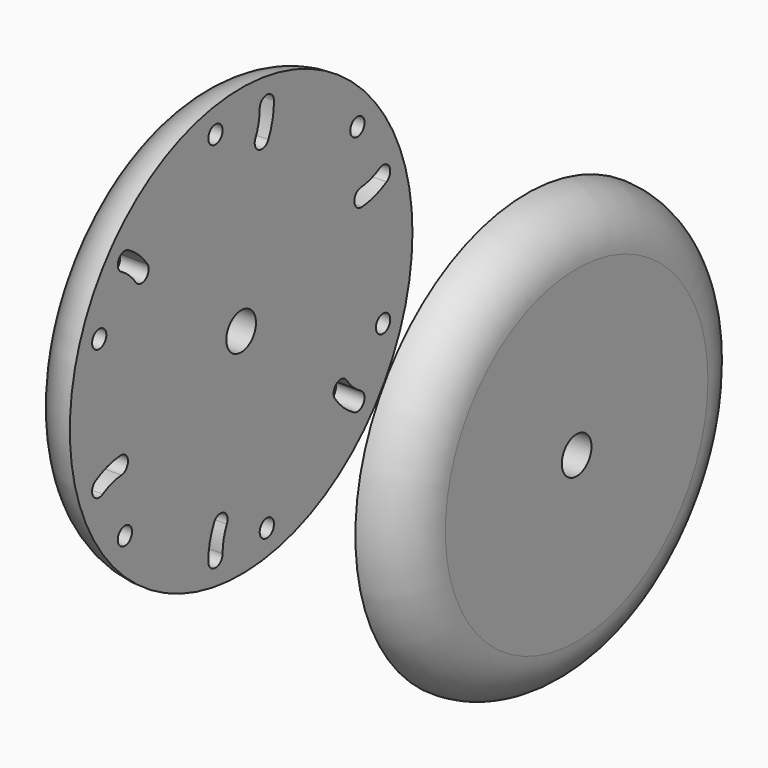
from build123d import *

# Parameters (mm, degrees)
F0_R     = 38.1
F1_DEPTH = 8.89
F2_R     = 8.88999
F3_R     = 3.302
F4_DEPTH = 8.89
F5_R     = 1.5875
F6_DEPTH = 5.08


# Not quite as in the source:
# - a fillet or chamfer is up to 0.001 mm smaller than in the source, because OpenCascade refuses the exact size


with BuildPart() as f1:
    # F0 (on Right) → F1 (new body)
    with BuildSketch(Plane.YZ):
        Circle(F0_R)
    extrude(amount=F1_DEPTH)

    # F2 (radius 8.89 in the source; OpenCascade refuses exactly that, so slightly less here)
    f2_edges = [f1.edges().sort_by_distance(p)[0] for p in [
        (8.89, -38.1, 0),
    ]]
    fillet(f2_edges, radius=F2_R)

    # F3 (on face) → F4 (cut)
    with BuildSketch(Plane.YZ.offset(8.89)):
        Circle(F3_R)
    extrude(amount=-F4_DEPTH, mode=Mode.SUBTRACT)

    # F5 (on face) → F6 (cut)
    with BuildSketch(Plane(origin=(0, 0, 0), x_dir=(0, -1, 0), z_dir=(-1, 0, 0))):
        with Locations((5.715, 33.1496630312)):
            Circle(F5_R)
        with BuildLine():
            ThreePointArc((-5.6047569444, 31.5659955413), (-4.5541453363, 32.0668090708), (-4.1275, 33.1496630312))
            ThreePointArc((-4.1275, 33.1496630312), (-5.715, 34.7371630312), (-7.3025, 33.1496630312))
            ThreePointArc((-7.3025, 33.1496630312), (-6.7978539604, 31.9888083675), (-5.6047569444, 31.5659955413))
        make_face()
        with BuildLine():
            ThreePointArc((-3.1712978707, 28.9178175232), (-3.8854737654, 30.9803982412), (-4.1275, 33.1496630312))
            ThreePointArc((-4.1275, 33.1496630312), (-4.5541453363, 32.0668090708), (-5.6047569444, 31.5659955413))
            ThreePointArc((-5.6047569444, 31.5659955413), (-5.433937276, 30.6305168235), (-5.1859467295, 29.712475169))
            ThreePointArc((-5.1859467295, 29.712475169), (-4.0220744225, 29.712032986), (-3.1712978707, 28.9178175232))
        make_face()
        with BuildLine():
            ThreePointArc((-5.6047569444, 31.5659955413), (-6.7978539604, 31.9888083675), (-7.3025, 33.1496630312))
            ThreePointArc((-7.3025, 33.1496630312), (-6.9824007866, 30.2806354058), (-6.0378455709, 27.552706069))
            ThreePointArc((-6.0378455709, 27.552706069), (-6.0813429107, 28.8177590943), (-5.1859467295, 29.712475169))
            ThreePointArc((-5.1859467295, 29.712475169), (-5.433937276, 30.6305168235), (-5.6047569444, 31.5659955413))
        make_face()
        with BuildLine():
            ThreePointArc((-3.0170717208, 28.2352617961), (-3.0561082102, 28.5851432138), (-3.1712978707, 28.9178175232))
            ThreePointArc((-3.1712978707, 28.9178175232), (-4.0220744225, 29.712032986), (-5.1859467295, 29.712475169))
            ThreePointArc((-5.1859467295, 29.712475169), (-6.0813429107, 28.8177590943), (-6.0378455709, 27.552706069))
            ThreePointArc((-6.0378455709, 27.552706069), (-4.254690303, 26.6867982855), (-3.0170717208, 28.2352617961))
        make_face()
        with BuildLine():
            ThreePointArc((-26.6292135324, 11.7124842426), (-28.772548779, 12.125280134), (-30.7722003119, 13.0003116615))
            ThreePointArc((-30.7722003119, 13.0003116615), (-30.1911349834, 12.419246333), (-29.9784503119, 11.625496333))
            ThreePointArc((-29.9784503119, 11.625496333), (-30.7722003119, 10.2506810045), (-32.3597003119, 10.2506810045))
            ThreePointArc((-32.3597003119, 10.2506810045), (-29.7149998974, 9.0933812423), (-26.8802661842, 8.547425386))
            ThreePointArc((-26.8802661842, 8.547425386), (-28.3372692866, 10.2554811402), (-26.6292135324, 11.7124842426))
        make_face()
        with BuildLine():
            ThreePointArc((-29.9784503119, 11.625496333), (-30.1911349834, 12.419246333), (-30.7722003119, 13.0003116615))
            ThreePointArc((-30.7722003119, 13.0003116615), (-32.9407656404, 12.419246333), (-32.3597003119, 10.2506810045))
            ThreePointArc((-32.3597003119, 10.2506810045), (-30.7722003119, 10.2506810045), (-29.9784503119, 11.625496333))
        make_face()
        with BuildLine():
            ThreePointArc((-25.1672398583, 10.1299548143), (-25.5886718302, 11.2071927657), (-26.6292135324, 11.7124842426))
            ThreePointArc((-26.6292135324, 11.7124842426), (-28.3372692866, 10.2554811402), (-26.8802661842, 8.547425386))
            ThreePointArc((-26.8802661842, 8.547425386), (-25.6775019069, 8.9638867862), (-25.1672398583, 10.1299548143))
        make_face()
        with Locations((-25.8509503119, 21.5241666982)):
            Circle(F5_R)
        with BuildLine():
            ThreePointArc((-23.4579156617, -17.2053332806), (-24.8870750135, -18.8551181072), (-26.6447003119, -20.1493513697))
            ThreePointArc((-26.6447003119, -20.1493513697), (-25.0572003119, -20.1493513697), (-24.2634503119, -21.5241666982))
            ThreePointArc((-24.2634503119, -21.5241666982), (-24.4761349834, -22.3179166982), (-25.0572003119, -22.8989820267))
            ThreePointArc((-25.0572003119, -22.8989820267), (-22.7325991108, -21.1872541634), (-20.8424206133, -19.005280683))
            ThreePointArc((-20.8424206133, -19.005280683), (-23.0501418387, -19.413054506), (-23.4579156617, -17.2053332806))
        make_face()
        with BuildLine():
            ThreePointArc((-24.2634503119, -21.5241666982), (-25.0572003119, -20.1493513697), (-26.6447003119, -20.1493513697))
            ThreePointArc((-26.6447003119, -20.1493513697), (-27.2257656404, -22.3179166982), (-25.0572003119, -22.8989820267))
            ThreePointArc((-25.0572003119, -22.8989820267), (-24.4761349834, -22.3179166982), (-24.2634503119, -21.5241666982))
        make_face()
        with BuildLine():
            ThreePointArc((-20.5626681375, -18.1053069818), (-21.6789425783, -16.5893575359), (-23.4579156617, -17.2053332806))
            ThreePointArc((-23.4579156617, -17.2053332806), (-23.0501418387, -19.413054506), (-20.8424206133, -19.005280683))
            ThreePointArc((-20.8424206133, -19.005280683), (-20.6342186917, -18.576532541), (-20.5626681375, -18.1053069818))
        make_face()
        with Locations((-31.5659503119, -11.625496333)):
            Circle(F5_R)
        with BuildLine():
            ThreePointArc((3.1712978707, -28.9178175232), (3.8854737654, -30.9803982412), (4.1275, -33.1496630312))
            ThreePointArc((4.1275, -33.1496630312), (5.715, -31.5621630312), (7.3025, -33.1496630312))
            ThreePointArc((7.3025, -33.1496630312), (6.9824007866, -30.2806354058), (6.0378455709, -27.552706069))
            ThreePointArc((6.0378455709, -27.552706069), (6.1530352313, -27.8853803783), (6.1920717208, -28.2352617961))
            ThreePointArc((6.1920717208, -28.2352617961), (4.9544531385, -29.7837253066), (3.1712978707, -28.9178175232))
        make_face()
        with BuildLine():
            ThreePointArc((7.3025, -33.1496630312), (5.715, -31.5621630312), (4.1275, -33.1496630312))
            ThreePointArc((4.1275, -33.1496630312), (5.715, -34.7371630312), (7.3025, -33.1496630312))
        make_face()
        with BuildLine():
            ThreePointArc((6.0378455709, -27.552706069), (3.9220159937, -26.801987946), (3.1712978707, -28.9178175232))
            ThreePointArc((3.1712978707, -28.9178175232), (4.9544531385, -29.7837253066), (6.1920717208, -28.2352617961))
            ThreePointArc((6.1920717208, -28.2352617961), (6.1530352313, -27.8853803783), (6.0378455709, -27.552706069))
        make_face()
        with Locations((-5.715, -33.1496630312)):
            Circle(F5_R)
        with BuildLine():
            ThreePointArc((26.6292135324, -11.7124842426), (28.772548779, -12.125280134), (30.7722003119, -13.0003116615))
            ThreePointArc((30.7722003119, -13.0003116615), (30.1911349834, -10.831746333), (32.3597003119, -10.2506810045))
            ThreePointArc((32.3597003119, -10.2506810045), (29.7149998974, -9.0933812423), (26.8802661842, -8.547425386))
            ThreePointArc((26.8802661842, -8.547425386), (27.9208078864, -9.052716863), (28.3422398583, -10.1299548143))
            ThreePointArc((28.3422398583, -10.1299548143), (27.8319778096, -11.2960228424), (26.6292135324, -11.7124842426))
        make_face()
        with BuildLine():
            ThreePointArc((32.3597003119, -10.2506810045), (30.1911349834, -10.831746333), (30.7722003119, -13.0003116615))
            ThreePointArc((30.7722003119, -13.0003116615), (32.3597003119, -13.0003116615), (33.1534503119, -11.625496333))
            ThreePointArc((33.1534503119, -11.625496333), (32.9407656404, -10.831746333), (32.3597003119, -10.2506810045))
        make_face()
        with BuildLine():
            ThreePointArc((26.8802661842, -8.547425386), (25.17221043, -10.0044284884), (26.6292135324, -11.7124842426))
            ThreePointArc((26.6292135324, -11.7124842426), (27.8319778096, -11.2960228424), (28.3422398583, -10.1299548143))
            ThreePointArc((28.3422398583, -10.1299548143), (27.9208078864, -9.052716863), (26.8802661842, -8.547425386))
        make_face()
        with Locations((25.8509503119, -21.5241666982)):
            Circle(F5_R)
        with BuildLine():
            ThreePointArc((23.4579156617, 17.2053332806), (24.8870750135, 18.8551181072), (26.6447003119, 20.1493513697))
            ThreePointArc((26.6447003119, 20.1493513697), (24.4761349834, 20.7304166982), (25.0572003119, 22.8989820267))
            ThreePointArc((25.0572003119, 22.8989820267), (22.7325991108, 21.1872541634), (20.8424206133, 19.005280683))
            ThreePointArc((20.8424206133, 19.005280683), (22.6213936967, 19.6212564276), (23.7376681375, 18.1053069818))
            ThreePointArc((23.7376681375, 18.1053069818), (23.6661175834, 17.6340814226), (23.4579156617, 17.2053332806))
        make_face()
        with BuildLine():
            ThreePointArc((25.0572003119, 22.8989820267), (24.4761349834, 20.7304166982), (26.6447003119, 20.1493513697))
            ThreePointArc((26.6447003119, 20.1493513697), (27.2257656404, 20.7304166982), (27.4384503119, 21.5241666982))
            ThreePointArc((27.4384503119, 21.5241666982), (26.6447003119, 22.8989820267), (25.0572003119, 22.8989820267))
        make_face()
        with BuildLine():
            ThreePointArc((20.8424206133, 19.005280683), (21.2501944363, 16.7975594576), (23.4579156617, 17.2053332806))
            ThreePointArc((23.4579156617, 17.2053332806), (23.6661175834, 17.6340814226), (23.7376681375, 18.1053069818))
            ThreePointArc((23.7376681375, 18.1053069818), (22.6213936967, 19.6212564276), (20.8424206133, 19.005280683))
        make_face()
        with Locations((31.5659503119, 11.625496333)):
            Circle(F5_R)
    extrude(amount=-F6_DEPTH, mode=Mode.SUBTRACT)


with BuildPart() as f8_1:
    # F8: instance of F1
    add(f1.part.mirror(Plane.YZ.offset(-25.4)))


solid = Compound([f1.part, f8_1.part])
